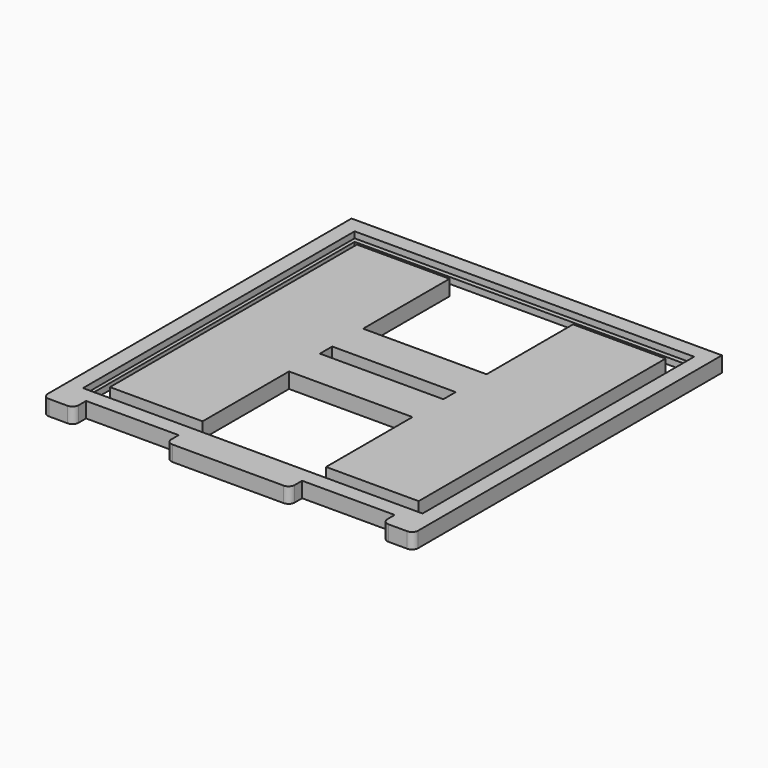
from build123d import *

# Parameters (mm, degrees)
F0_W     = 139.7
F0_H     = 139.7
F1_DEPTH = 6.35
F0_W_2   = 50.8
F0_H_2   = 6.35
F2_W     = 146.05
F2_H     = 1.27
F3_DEPTH = 149.225
F4_R     = 2.54


with BuildPart() as f1:
    # F0 (on Top) → F1 (new body)
    with BuildSketch(Plane.XY):
        Polygon((0, 158.75), (0, 0), (12.7, 0), (12.7, 6.35), (50.8, 6.35), (50.8, 0), (101.6, 0), (101.6, 6.35), (139.7, 6.35), (139.7, 0), (152.4, 0), (152.4, 158.75), align=None)
        with Locations((76.2, 82.55)):
            Rectangle(F0_W, F0_H, mode=Mode.SUBTRACT)
    extrude(amount=F1_DEPTH)

    # F2 (on face) → F3 (cut)
    with BuildSketch(Plane(origin=(0, 158.75, 0), x_dir=(-1, 0, 0), z_dir=(0, 1, 0))):
        with Locations((-76.2, 3.175)):
            Rectangle(F2_W, F2_H)
    extrude(amount=-F3_DEPTH, mode=Mode.SUBTRACT)

    # F4
    f4_edges = [f1.edges().sort_by_distance(p)[0] for p in [
        (12.7, 0, 3.175),
        (0, 0, 3.175),
        (50.8, 0, 3.175),
        (101.6, 0, 3.175),
        (139.7, 0, 3.175),
        (152.4, 0, 3.175),
    ]]
    fillet(f4_edges, radius=F4_R)


with BuildPart() as f1b:
    # F0 (on Top) → F1, piece 2 (new body)
    with BuildSketch(Plane.XY):
        Polygon((50.8, 145.6505734556), (12.7, 145.6505734556), (12.7, 18.6505734556), (50.8, 18.6505734556), (50.8, 63.1005734556), (101.6, 63.1005734556), (101.6, 18.6505734556), (139.7, 18.6505734556), (139.7, 145.6505734556), (101.6, 145.6505734556), (101.6, 101.2005734556), (50.8, 101.2005734556), align=None)
        with Locations((76.2, 82.1505734556)):
            Rectangle(F0_W_2, F0_H_2, mode=Mode.SUBTRACT)
    extrude(amount=F1_DEPTH)


solid = Compound([f1.part, f1b.part])
